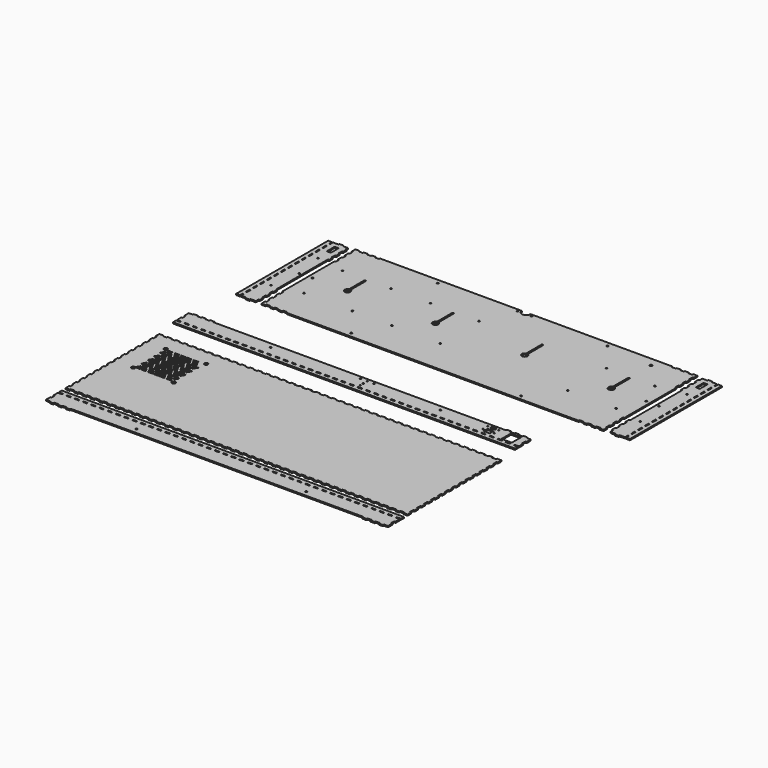
from build123d import *

# Parameters (mm, degrees)
F0_R     = 4.572
F1_DEPTH = 3.175
F0_R_2   = 2.1828252
F0_R_3   = 2.0447
F0_R_4   = 3.175
F0_W     = 2.9972
F0_H     = 11.8654322
F0_R_5   = 2.0828
F0_H_2   = 11.8654068
F0_H_3   = 11.8654576
F0_W_2   = 10.4902
F0_H_4   = 25.4
F0_W_3   = 10.7526836
F0_H_5   = 2.9972
F0_W_4   = 10.7526582
F0_R_6   = 1.5875
F0_W_5   = 16.002
F0_H_6   = 13.3096
F0_R_7   = 1.4224
F0_W_6   = 13.0048
F0_H_7   = 4.699
F0_W_7   = 26.67
F0_H_8   = 30.988


# Not quite as in the source:
# - ends of sketch curves that miss each other by under 0.0002 mm in the source are joined
# - a length typed as a fraction of an inch, garbled in the dataset ("3 / 203.2 mm" for 3/8 in), is restored


with BuildPart() as f1:
    # F0 (on Top) → F1 (new body)
    with BuildSketch(Plane.XY):
        Polygon((-501.14835, -83.3475346), (-511.9010082, -83.3475346), (-511.9010082, -95.2129668), (-508.9038082, -95.2129668), (-508.9038082, -105.8809668), (-511.9010082, -105.8809668), (-511.9010082, -117.746399), (-508.9038082, -117.746399), (-508.9038082, -128.4143736), (-511.9010082, -128.4143736), (-511.9010082, -140.2798058), (-508.9038082, -140.2798058), (-508.9038082, -150.9478058), (-511.9010082, -150.9478058), (-511.9010082, -162.813238), (-508.9038082, -162.813238), (-508.9038082, -173.481238), (-511.9010082, -173.481238), (-511.9010082, -185.3466702), (-508.9038082, -185.3466702), (-508.9038082, -196.0146702), (-511.9010082, -196.0146702), (-511.9010082, -207.8801024), (-508.9038082, -207.8801024), (-508.9038082, -218.5481024), (-511.9010082, -218.5481024), (-511.9010082, -230.4135346), (-508.9038082, -230.4135346), (-508.9038082, -241.0815346), (-511.9010082, -241.0815346), (-511.9010082, -252.9469668), (-508.9038082, -252.9469668), (-508.9038082, -263.6149668), (-511.9010082, -263.6149668), (-511.9010082, -275.4803736), (-508.9038082, -275.4803736), (-508.9038082, -286.1483736), (-511.9010082, -286.1483736), (-511.9010082, -298.0138312), (-508.9038082, -298.0138312), (-508.9038082, -308.6818312), (-511.9010082, -308.6818312), (-511.9010082, -320.547238), (-508.9038082, -320.547238), (-508.9038082, -331.215238), (-511.9010082, -331.215238), (-511.9010082, -343.0806702), (-508.9038082, -343.0806702), (-508.9038082, -353.7486702), (-511.9010082, -353.7486702), (-511.9010082, -365.614077), (-508.9038082, -365.614077), (-508.9038082, -376.282077), (-511.9010082, -376.282077), (-511.9010082, -388.1475346), (-501.14835, -388.1475346), (-501.14835, -385.1503346), (-490.48035, -385.1503346), (-490.48035, -388.1475346), (-479.7276918, -388.1475346), (-479.7276918, -385.1503346), (-469.0596918, -385.1503346), (-469.0596918, -388.1475346), (-458.3070082, -388.1475346), (-458.3070082, -385.1503346), (-447.6390082, -385.1503346), (-447.6390082, -388.1475346), (-436.88635, -388.1475346), (-436.88635, -385.1503346), (-426.21835, -385.1503346), (-426.21835, -388.1475346), (-415.4656918, -388.1475346), (-415.4656918, -385.1503346), (-404.7976918, -385.1503346), (-404.7976918, -388.1475346), (-394.0450082, -388.1475346), (-394.0450082, -385.1503346), (-383.3770082, -385.1503346), (-383.3770082, -388.1475346), (-372.62435, -388.1475346), (-372.62435, -385.1503346), (-361.95635, -385.1503346), (-361.95635, -388.1475346), (-351.2036918, -388.1475346), (-351.2036918, -385.1503346), (-340.5356918, -385.1503346), (-340.5356918, -388.1475346), (-329.7830082, -388.1475346), (-329.7830082, -385.1503346), (-319.1150082, -385.1503346), (-319.1150082, -388.1475346), (-308.36235, -388.1475346), (-308.36235, -385.1503346), (-297.69435, -385.1503346), (-297.69435, -388.1475346), (-286.9416918, -388.1475346), (-286.9416918, -385.1503346), (-276.2736918, -385.1503346), (-276.2736918, -388.1475346), (-265.5210082, -388.1475346), (-265.5210082, -385.1503346), (-254.8530082, -385.1503346), (-254.8530082, -388.1475346), (-244.10035, -388.1475346), (-244.10035, -385.1503346), (-233.43235, -385.1503346), (-233.43235, -388.1475346), (-222.6796918, -388.1475346), (-222.6796918, -385.1503346), (-212.0116918, -385.1503346), (-212.0116918, -388.1475346), (-201.2590082, -388.1475346), (-201.2590082, -385.1503346), (-190.5910082, -385.1503346), (-190.5910082, -388.1475346), (-179.83835, -388.1475346), (-179.83835, -385.1503346), (-169.17035, -385.1503346), (-169.17035, -388.1475346), (-158.4176918, -388.1475346), (-158.4176918, -385.1503346), (-147.7496918, -385.1503346), (-147.7496918, -388.1475346), (-136.9970082, -388.1475346), (-136.9970082, -385.1503346), (-126.3290082, -385.1503346), (-126.3290082, -388.1475346), (-115.57635, -388.1475346), (-115.57635, -385.1503346), (-104.90835, -385.1503346), (-104.90835, -388.1475346), (-94.1556918, -388.1475346), (-94.1556918, -385.1503346), (-83.4876918, -385.1503346), (-83.4876918, -388.1475346), (-72.7350082, -388.1475346), (-72.7350082, -385.1503346), (-62.0670082, -385.1503346), (-62.0670082, -388.1475346), (-51.31435, -388.1475346), (-51.31435, -385.1503346), (-40.64635, -385.1503346), (-40.64635, -388.1475346), (-29.8936918, -388.1475346), (-29.8936918, -385.1503346), (-19.2256918, -385.1503346), (-19.2256918, -388.1475346), (-8.4730082, -388.1475346), (-8.4730082, -385.1503346), (2.1949918, -385.1503346), (2.1949918, -388.1475346), (12.94765, -388.1475346), (12.94765, -385.1503346), (23.61565, -385.1503346), (23.61565, -388.1475346), (34.3683082, -388.1475346), (34.3683082, -385.1503346), (45.0363082, -385.1503346), (45.0363082, -388.1475346), (55.7889918, -388.1475346), (55.7889918, -385.1503346), (66.4569918, -385.1503346), (66.4569918, -388.1475346), (77.20965, -388.1475346), (77.20965, -385.1503346), (87.87765, -385.1503346), (87.87765, -388.1475346), (98.6303082, -388.1475346), (98.6303082, -385.1503346), (109.2983082, -385.1503346), (109.2983082, -388.1475346), (120.0509918, -388.1475346), (120.0509918, -385.1503346), (130.7189918, -385.1503346), (130.7189918, -388.1475346), (141.47165, -388.1475346), (141.47165, -385.1503346), (152.13965, -385.1503346), (152.13965, -388.1475346), (162.8923082, -388.1475346), (162.8923082, -385.1503346), (173.5603082, -385.1503346), (173.5603082, -388.1475346), (184.3129918, -388.1475346), (184.3129918, -385.1503346), (194.9809918, -385.1503346), (194.9809918, -388.1475346), (205.73365, -388.1475346), (205.73365, -385.1503346), (216.40165, -385.1503346), (216.40165, -388.1475346), (227.1543082, -388.1475346), (227.1543082, -385.1503346), (237.8223082, -385.1503346), (237.8223082, -388.1475346), (248.5749918, -388.1475346), (248.5749918, -385.1503346), (259.2429918, -385.1503346), (259.2429918, -388.1475346), (269.99565, -388.1475346), (269.99565, -385.1503346), (280.66365, -385.1503346), (280.66365, -388.1475346), (291.4163082, -388.1475346), (291.4163082, -385.1503346), (302.0843082, -385.1503346), (302.0843082, -388.1475346), (312.8369918, -388.1475346), (312.8369918, -385.1503346), (323.5049918, -385.1503346), (323.5049918, -388.1475346), (334.25765, -388.1475346), (334.25765, -385.1503346), (344.92565, -385.1503346), (344.92565, -388.1475346), (355.6783082, -388.1475346), (355.6783082, -385.1503346), (366.3463082, -385.1503346), (366.3463082, -388.1475346), (377.0989918, -388.1475346), (377.0989918, -376.282077), (374.1017918, -376.282077), (374.1017918, -365.614077), (377.0989918, -365.614077), (377.0989918, -353.7486702), (374.1017918, -353.7486702), (374.1017918, -343.0806702), (377.0989918, -343.0806702), (377.0989918, -331.215238), (374.1017918, -331.215238), (374.1017918, -320.547238), (377.0989918, -320.547238), (377.0989918, -308.6818312), (374.1017918, -308.6818312), (374.1017918, -298.0138312), (377.0989918, -298.0138312), (377.0989918, -286.1483736), (374.1017918, -286.1483736), (374.1017918, -275.4803736), (377.0989918, -275.4803736), (377.0989918, -263.6149668), (374.1017918, -263.6149668), (374.1017918, -252.9469668), (377.0989918, -252.9469668), (377.0989918, -241.0815346), (374.1017918, -241.0815346), (374.1017918, -230.4135346), (377.0989918, -230.4135346), (377.0989918, -218.5481024), (374.1017918, -218.5481024), (374.1017918, -207.8801024), (377.0989918, -207.8801024), (377.0989918, -196.0146702), (374.1017918, -196.0146702), (374.1017918, -185.3466702), (377.0989918, -185.3466702), (377.0989918, -173.481238), (374.1017918, -173.481238), (374.1017918, -162.813238), (377.0989918, -162.813238), (377.0989918, -150.9478058), (374.1017918, -150.9478058), (374.1017918, -140.2798058), (377.0989918, -140.2798058), (377.0989918, -128.4143736), (374.1017918, -128.4143736), (374.1017918, -117.746399), (377.0989918, -117.746399), (377.0989918, -105.8809668), (374.1017918, -105.8809668), (374.1017918, -95.2129668), (377.0989918, -95.2129668), (377.0989918, -83.3475346), (366.3463082, -83.3475346), (366.3463082, -86.3447346), (355.6783082, -86.3447346), (355.6783082, -83.3475346), (344.92565, -83.3475346), (344.92565, -86.3447346), (334.25765, -86.3447346), (334.25765, -83.3475346), (323.5049918, -83.3475346), (323.5049918, -86.3447346), (312.8369918, -86.3447346), (312.8369918, -83.3475346), (302.0843082, -83.3475346), (302.0843082, -86.3447346), (291.4163082, -86.3447346), (291.4163082, -83.3475346), (280.66365, -83.3475346), (280.66365, -86.3447346), (269.99565, -86.3447346), (269.99565, -83.3475346), (259.2429918, -83.3475346), (259.2429918, -86.3447346), (248.5749918, -86.3447346), (248.5749918, -83.3475346), (237.8223082, -83.3475346), (237.8223082, -86.3447346), (227.1543082, -86.3447346), (227.1543082, -83.3475346), (216.40165, -83.3475346), (216.40165, -86.3447346), (205.73365, -86.3447346), (205.73365, -83.3475346), (194.9809918, -83.3475346), (194.9809918, -86.3447346), (184.3129918, -86.3447346), (184.3129918, -83.3475346), (173.5603082, -83.3475346), (173.5603082, -86.3447346), (162.8923082, -86.3447346), (162.8923082, -83.3475346), (152.13965, -83.3475346), (152.13965, -86.3447346), (141.47165, -86.3447346), (141.47165, -83.3475346), (130.7189918, -83.3475346), (130.7189918, -86.3447346), (120.0509918, -86.3447346), (120.0509918, -83.3475346), (109.2983082, -83.3475346), (109.2983082, -86.3447346), (98.6303082, -86.3447346), (98.6303082, -83.3475346), (87.87765, -83.3475346), (87.87765, -86.3447346), (77.20965, -86.3447346), (77.20965, -83.3475346), (66.4569918, -83.3475346), (66.4569918, -86.3447346), (55.7889918, -86.3447346), (55.7889918, -83.3475346), (45.0363082, -83.3475346), (45.0363082, -86.3447346), (34.3683082, -86.3447346), (34.3683082, -83.3475346), (23.61565, -83.3475346), (23.61565, -86.3447346), (12.94765, -86.3447346), (12.94765, -83.3475346), (2.1949918, -83.3475346), (2.1949918, -86.3447346), (-8.4730082, -86.3447346), (-8.4730082, -83.3475346), (-19.2256918, -83.3475346), (-19.2256918, -86.3447346), (-29.8936918, -86.3447346), (-29.8936918, -83.3475346), (-40.64635, -83.3475346), (-40.64635, -86.3447346), (-51.31435, -86.3447346), (-51.31435, -83.3475346), (-62.0670082, -83.3475346), (-62.0670082, -86.3447346), (-72.7350082, -86.3447346), (-72.7350082, -83.3475346), (-83.4876918, -83.3475346), (-83.4876918, -86.3447346), (-94.1556918, -86.3447346), (-94.1556918, -83.3475346), (-104.90835, -83.3475346), (-104.90835, -86.3447346), (-115.57635, -86.3447346), (-115.57635, -83.3475346), (-126.3290082, -83.3475346), (-126.3290082, -86.3447346), (-136.9970082, -86.3447346), (-136.9970082, -83.3475346), (-147.7496918, -83.3475346), (-147.7496918, -86.3447346), (-158.4176918, -86.3447346), (-158.4176918, -83.3475346), (-169.17035, -83.3475346), (-169.17035, -86.3447346), (-179.83835, -86.3447346), (-179.83835, -83.3475346), (-190.5910082, -83.3475346), (-190.5910082, -86.3447346), (-201.2590082, -86.3447346), (-201.2590082, -83.3475346), (-212.0116918, -83.3475346), (-212.0116918, -86.3447346), (-222.6796918, -86.3447346), (-222.6796918, -83.3475346), (-233.43235, -83.3475346), (-233.43235, -86.3447346), (-244.10035, -86.3447346), (-244.10035, -83.3475346), (-254.8530082, -83.3475346), (-254.8530082, -86.3447346), (-265.5210082, -86.3447346), (-265.5210082, -83.3475346), (-276.2736918, -83.3475346), (-276.2736918, -86.3447346), (-286.9416918, -86.3447346), (-286.9416918, -83.3475346), (-297.69435, -83.3475346), (-297.69435, -86.3447346), (-308.36235, -86.3447346), (-308.36235, -83.3475346), (-319.1150082, -83.3475346), (-319.1150082, -86.3447346), (-329.7830082, -86.3447346), (-329.7830082, -83.3475346), (-340.5356918, -83.3475346), (-340.5356918, -86.3447346), (-351.2036918, -86.3447346), (-351.2036918, -83.3475346), (-361.95635, -83.3475346), (-361.95635, -86.3447346), (-372.62435, -86.3447346), (-372.62435, -83.3475346), (-383.3770082, -83.3475346), (-383.3770082, -86.3447346), (-394.0450082, -86.3447346), (-394.0450082, -83.3475346), (-404.7976918, -83.3475346), (-404.7976918, -86.3447346), (-415.4656918, -86.3447346), (-415.4656918, -83.3475346), (-426.21835, -83.3475346), (-426.21835, -86.3447346), (-436.88635, -86.3447346), (-436.88635, -83.3475346), (-447.6390082, -83.3475346), (-447.6390082, -86.3447346), (-458.3070082, -86.3447346), (-458.3070082, -83.3475346), (-469.0596918, -83.3475346), (-469.0596918, -86.3447346), (-479.7276918, -86.3447346), (-479.7276918, -83.3475346), (-490.48035, -83.3475346), (-490.48035, -86.3447346), (-501.14835, -86.3447346), align=None)
        with Locations((-355.68255, -231.9860994)):
            Circle(F0_R, mode=Mode.SUBTRACT)
        with BuildLine():
            ThreePointArc((-457.6334996089, -228.582496957), (-456.511230744, -230.1224381631), (-456.11415, -231.9860994))
            ThreePointArc((-456.11415, -231.9860994), (-464.4699540022, -234.5524219192), (-458.9951698043, -227.7383035036))
            Line((-458.9951698043, -227.7383035036), (-452.8834732, -217.1524994))
            Line((-452.8834732, -217.1524994), (-446.28435, -228.5824994))
            Line((-446.28435, -228.5824994), (-457.6334996089, -228.582496957))
        make_face(mode=Mode.SUBTRACT)
        Polygon((-438.66435, -210.8024994), (-445.2634732, -222.2324994), (-451.862571, -210.8024994), align=None, mode=Mode.SUBTRACT)
        Polygon((-444.242571, -228.5824994), (-437.6434732, -217.1524994), (-431.04435, -228.5824994), align=None, mode=Mode.SUBTRACT)
        Polygon((-420.88435, -210.8024994), (-427.4834732, -222.2324994), (-434.082571, -210.8024994), align=None, mode=Mode.SUBTRACT)
        Polygon((-459.482571, -208.2624994), (-452.8834732, -196.8324994), (-446.28435, -208.2624994), align=None, mode=Mode.SUBTRACT)
        Polygon((-444.242571, -208.2624994), (-437.6434732, -196.8324994), (-431.04435, -208.2624994), align=None, mode=Mode.SUBTRACT)
        Polygon((-426.462571, -228.5824994), (-419.8634732, -217.1524994), (-413.26435, -228.5824994), align=None, mode=Mode.SUBTRACT)
        Polygon((-405.64435, -210.8024994), (-412.2434732, -222.2324994), (-418.842571, -210.8024994), align=None, mode=Mode.SUBTRACT)
        Polygon((-410.9734732, -228.5824994), (-404.37435, -217.1524994), (-397.7752268, -228.5824994), align=None, mode=Mode.SUBTRACT)
        Polygon((-390.1552268, -210.8024994), (-396.75435, -222.2324994), (-403.3534732, -210.8024994), align=None, mode=Mode.SUBTRACT)
        Polygon((-426.462571, -208.2624994), (-419.8634732, -196.8324994), (-413.26435, -208.2624994), align=None, mode=Mode.SUBTRACT)
        Polygon((-410.9734732, -208.2624994), (-404.37435, -196.8324994), (-397.7752268, -208.2624994), align=None, mode=Mode.SUBTRACT)
        Polygon((-438.66435, -190.4824994), (-445.2634732, -201.9124994), (-451.862571, -190.4824994), align=None, mode=Mode.SUBTRACT)
        Polygon((-420.88435, -190.4824994), (-427.4834732, -201.9124994), (-434.082571, -190.4824994), align=None, mode=Mode.SUBTRACT)
        Polygon((-459.482571, -187.9424994), (-452.8834732, -176.5124994), (-446.28435, -187.9424994), align=None, mode=Mode.SUBTRACT)
        Polygon((-438.66435, -170.1624994), (-445.2634732, -181.5924994), (-451.862571, -170.1624994), align=None, mode=Mode.SUBTRACT)
        Polygon((-444.242571, -187.9424994), (-437.6434732, -176.5124994), (-431.04435, -187.9424994), align=None, mode=Mode.SUBTRACT)
        Polygon((-420.88435, -170.1624994), (-427.4834732, -181.5924994), (-434.082571, -170.1624994), align=None, mode=Mode.SUBTRACT)
        Polygon((-405.64435, -190.4824994), (-412.2434732, -201.9124994), (-418.842571, -190.4824994), align=None, mode=Mode.SUBTRACT)
        Polygon((-390.1552268, -190.4824994), (-396.75435, -201.9124994), (-403.3534732, -190.4824994), align=None, mode=Mode.SUBTRACT)
        Polygon((-426.462571, -187.9424994), (-419.8634732, -176.5124994), (-413.26435, -187.9424994), align=None, mode=Mode.SUBTRACT)
        Polygon((-405.64435, -170.1624994), (-412.2434732, -181.5924994), (-418.842571, -170.1624994), align=None, mode=Mode.SUBTRACT)
        Polygon((-410.9734732, -187.9424994), (-404.37435, -176.5124994), (-397.7752268, -187.9424994), align=None, mode=Mode.SUBTRACT)
        Polygon((-390.1552268, -170.1624994), (-396.75435, -181.5924994), (-403.3534732, -170.1624994), align=None, mode=Mode.SUBTRACT)
        with Locations((-460.68615, -126.9824994)):
            Circle(F0_R, mode=Mode.SUBTRACT)
        Polygon((-459.482571, -167.6224994), (-452.8834732, -156.1924994), (-446.28435, -167.6224994), align=None, mode=Mode.SUBTRACT)
        Polygon((-444.242571, -167.6224994), (-437.6434732, -156.1924994), (-431.04435, -167.6224994), align=None, mode=Mode.SUBTRACT)
        Polygon((-438.66435, -149.8424994), (-445.2634732, -161.2724994), (-451.862571, -149.8424994), align=None, mode=Mode.SUBTRACT)
        Polygon((-420.88435, -149.8424994), (-427.4834732, -161.2724994), (-434.082571, -149.8424994), align=None, mode=Mode.SUBTRACT)
        Polygon((-426.462571, -167.6224994), (-419.8634732, -156.1924994), (-413.26435, -167.6224994), align=None, mode=Mode.SUBTRACT)
        Polygon((-410.9734732, -167.6224994), (-404.37435, -156.1924994), (-397.7752268, -167.6224994), align=None, mode=Mode.SUBTRACT)
        Polygon((-405.64435, -149.8424994), (-412.2434732, -161.2724994), (-418.842571, -149.8424994), align=None, mode=Mode.SUBTRACT)
        Polygon((-390.1552268, -149.8424994), (-396.75435, -161.2724994), (-403.3534732, -149.8424994), align=None, mode=Mode.SUBTRACT)
        Polygon((-459.482571, -147.3024994), (-452.8834732, -135.8724994), (-446.28435, -147.3024994), align=None, mode=Mode.SUBTRACT)
        Polygon((-438.66435, -129.5224994), (-445.2634732, -140.9524994), (-451.862571, -129.5224994), align=None, mode=Mode.SUBTRACT)
        Polygon((-444.242571, -147.3024994), (-437.6434732, -135.8724994), (-431.04435, -147.3024994), align=None, mode=Mode.SUBTRACT)
        Polygon((-420.88435, -129.5224994), (-427.4834732, -140.9524994), (-434.082571, -129.5224994), align=None, mode=Mode.SUBTRACT)
        Polygon((-426.462571, -147.3024994), (-419.8634732, -135.8724994), (-413.26435, -147.3024994), align=None, mode=Mode.SUBTRACT)
        Polygon((-405.64435, -129.5224994), (-412.2434732, -140.9524994), (-418.842571, -129.5224994), align=None, mode=Mode.SUBTRACT)
        Polygon((-410.9734732, -147.3024994), (-404.37435, -135.8724994), (-397.7752268, -147.3024994), align=None, mode=Mode.SUBTRACT)
        Polygon((-390.1552268, -129.5224994), (-396.75435, -140.9524994), (-403.3534732, -129.5224994), align=None, mode=Mode.SUBTRACT)
        Polygon((-395.7334732, -228.5824994), (-389.13435, -217.1524994), (-382.5352268, -228.5824994), align=None, mode=Mode.SUBTRACT)
        Polygon((-372.3752268, -210.8024994), (-378.97435, -222.2324994), (-385.5734732, -210.8024994), align=None, mode=Mode.SUBTRACT)
        Polygon((-377.9534732, -228.5824994), (-371.35435, -217.1524994), (-364.7552268, -228.5824994), align=None, mode=Mode.SUBTRACT)
        Polygon((-357.1352268, -210.8024994), (-363.73435, -222.2324994), (-370.3334732, -210.8024994), align=None, mode=Mode.SUBTRACT)
        Polygon((-395.7334732, -208.2624994), (-389.13435, -196.8324994), (-382.5352268, -208.2624994), align=None, mode=Mode.SUBTRACT)
        Polygon((-377.9534732, -208.2624994), (-371.35435, -196.8324994), (-364.7552268, -208.2624994), align=None, mode=Mode.SUBTRACT)
        Polygon((-372.3752268, -190.4824994), (-378.97435, -201.9124994), (-385.5734732, -190.4824994), align=None, mode=Mode.SUBTRACT)
        Polygon((-357.1352268, -190.4824994), (-363.73435, -201.9124994), (-370.3334732, -190.4824994), align=None, mode=Mode.SUBTRACT)
        Polygon((-395.7334732, -187.9424994), (-389.13435, -176.5124994), (-382.5352268, -187.9424994), align=None, mode=Mode.SUBTRACT)
        Polygon((-372.3752268, -170.1624994), (-378.97435, -181.5924994), (-385.5734732, -170.1624994), align=None, mode=Mode.SUBTRACT)
        Polygon((-377.9534732, -187.9424994), (-371.35435, -176.5124994), (-364.7552268, -187.9424994), align=None, mode=Mode.SUBTRACT)
        Polygon((-357.1352268, -170.1624994), (-363.73435, -181.5924994), (-370.3334732, -170.1624994), align=None, mode=Mode.SUBTRACT)
        Polygon((-395.7334732, -167.6224994), (-389.13435, -156.1924994), (-382.5352268, -167.6224994), align=None, mode=Mode.SUBTRACT)
        Polygon((-377.9534732, -167.6224994), (-371.35435, -156.1924994), (-364.7552268, -167.6224994), align=None, mode=Mode.SUBTRACT)
        Polygon((-372.3752268, -149.8424994), (-378.97435, -161.2724994), (-385.5734732, -149.8424994), align=None, mode=Mode.SUBTRACT)
        Polygon((-357.1352268, -149.8424994), (-363.73435, -161.2724994), (-370.3334732, -149.8424994), align=None, mode=Mode.SUBTRACT)
        Polygon((-395.7334732, -147.3024994), (-389.13435, -135.8724994), (-382.5352268, -147.3024994), align=None, mode=Mode.SUBTRACT)
        Polygon((-372.3752268, -129.5224994), (-378.97435, -140.9524994), (-385.5734732, -129.5224994), align=None, mode=Mode.SUBTRACT)
        Polygon((-377.9534732, -147.3024994), (-371.35435, -135.8724994), (-364.7552268, -147.3024994), align=None, mode=Mode.SUBTRACT)
        with BuildLine():
            ThreePointArc((-357.958210521, -130.9479190743), (-357.9737139071, -123.0260171302), (-351.11055, -126.9824994))
            ThreePointArc((-351.11055, -126.9824994), (-353.3913860929, -130.9389816698), (-357.958210521, -130.9479190743))
        make_face(mode=Mode.SUBTRACT)
    extrude(amount=F1_DEPTH)


with BuildPart() as f1b:
    # F0 (on Top) → F1, piece 2 (new body)
    with BuildSketch(Plane.XY):
        with BuildLine():
            Line((-369.32235, 150.7120684), (-358.5696664, 150.7120684))
            Line((-358.5696664, 150.7120684), (380.4009918, 150.7120684))
            Line((380.4009918, 150.7120684), (391.15365, 150.7120684))
            Line((391.15365, 150.7120684), (391.15365, 153.7092684))
            Line((391.15365, 153.7092684), (401.82165, 153.7092684))
            Line((401.82165, 153.7092684), (401.82165, 150.7120684))
            Line((401.82165, 150.7120684), (412.5743336, 150.7120684))
            Line((412.5743336, 150.7120684), (412.5743336, 153.7092684))
            Line((412.5743336, 153.7092684), (423.2423336, 153.7092684))
            Line((423.2423336, 153.7092684), (423.2423336, 150.7120684))
            Line((423.2423336, 150.7120684), (433.9949918, 150.7120684))
            Line((433.9949918, 150.7120684), (433.9949918, 153.7092684))
            Line((433.9949918, 153.7092684), (444.6629918, 153.7092684))
            Line((444.6629918, 153.7092684), (444.6629918, 150.7120684))
            Line((444.6629918, 150.7120684), (455.41565, 150.7120684))
            Line((455.41565, 150.7120684), (455.41565, 162.5775006))
            Line((455.41565, 162.5775006), (452.41845, 162.5775006))
            Line((452.41845, 162.5775006), (452.41845, 173.2455006))
            Line((452.41845, 173.2455006), (455.41565, 173.2455006))
            Line((455.41565, 173.2455006), (455.41565, 185.1109074))
            Line((455.41565, 185.1109074), (452.41845, 185.1109074))
            Line((452.41845, 185.1109074), (452.41845, 195.7789074))
            Line((452.41845, 195.7789074), (455.41565, 195.7789074))
            Line((455.41565, 195.7789074), (455.41565, 207.644365))
            Line((455.41565, 207.644365), (452.41845, 207.644365))
            Line((452.41845, 207.644365), (452.41845, 218.312365))
            Line((452.41845, 218.312365), (455.41565, 218.312365))
            Line((455.41565, 218.312365), (455.41565, 387.9117718))
            Line((455.41565, 387.9117718), (452.41845, 387.9117718))
            Line((452.41845, 387.9117718), (452.41845, 398.5797718))
            Line((452.41845, 398.5797718), (455.41565, 398.5797718))
            Line((455.41565, 398.5797718), (455.41565, 410.445204))
            Line((455.41565, 410.445204), (452.41845, 410.445204))
            Line((452.41845, 410.445204), (452.41845, 421.113204))
            Line((452.41845, 421.113204), (455.41565, 421.113204))
            Line((455.41565, 421.113204), (455.41565, 432.9786362))
            Line((455.41565, 432.9786362), (452.41845, 432.9786362))
            Line((452.41845, 432.9786362), (452.41845, 443.6466362))
            Line((452.41845, 443.6466362), (455.41565, 443.6466362))
            Line((455.41565, 443.6466362), (455.41565, 455.5120684))
            Line((455.41565, 455.5120684), (444.6629918, 455.5120684))
            Line((444.6629918, 455.5120684), (444.6629918, 452.5148684))
            Line((444.6629918, 452.5148684), (433.9949918, 452.5148684))
            Line((433.9949918, 452.5148684), (433.9949918, 455.5120684))
            Line((433.9949918, 455.5120684), (423.2423336, 455.5120684))
            Line((423.2423336, 455.5120684), (423.2423336, 452.5148684))
            Line((423.2423336, 452.5148684), (412.5743336, 452.5148684))
            Line((412.5743336, 452.5148684), (412.5743336, 455.5120684))
            Line((412.5743336, 455.5120684), (401.82165, 455.5120684))
            Line((401.82165, 455.5120684), (401.82165, 452.5148684))
            Line((401.82165, 452.5148684), (391.15365, 452.5148684))
            Line((391.15365, 452.5148684), (391.15365, 455.5120684))
            Line((391.15365, 455.5120684), (380.4009918, 455.5120684))
            Line((380.4009918, 455.5120684), (22.3456754, 455.5120684))
            ThreePointArc((22.3456754, 455.5120684), (10.91565, 444.0820684), (-0.51435, 455.5120684))
            Line((-0.51435, 455.5120684), (-358.5696664, 455.5120684))
            Line((-358.5696664, 455.5120684), (-369.32235, 455.5120684))
            Line((-369.32235, 455.5120684), (-369.32235, 452.5148684))
            Line((-369.32235, 452.5148684), (-379.99035, 452.5148684))
            Line((-379.99035, 452.5148684), (-379.99035, 455.5120684))
            Line((-379.99035, 455.5120684), (-390.7430082, 455.5120684))
            Line((-390.7430082, 455.5120684), (-390.7430082, 452.5148684))
            Line((-390.7430082, 452.5148684), (-401.4110082, 452.5148684))
            Line((-401.4110082, 452.5148684), (-401.4110082, 455.5120684))
            Line((-401.4110082, 455.5120684), (-412.1636664, 455.5120684))
            Line((-412.1636664, 455.5120684), (-412.1636664, 452.5148684))
            Line((-412.1636664, 452.5148684), (-422.8316664, 452.5148684))
            Line((-422.8316664, 452.5148684), (-422.8316664, 455.5120684))
            Line((-422.8316664, 455.5120684), (-433.58435, 455.5120684))
            Line((-433.58435, 455.5120684), (-433.58435, 443.6466362))
            Line((-433.58435, 443.6466362), (-430.58715, 443.6466362))
            Line((-430.58715, 443.6466362), (-430.58715, 432.9786362))
            Line((-430.58715, 432.9786362), (-433.58435, 432.9786362))
            Line((-433.58435, 432.9786362), (-433.58435, 421.113204))
            Line((-433.58435, 421.113204), (-430.58715, 421.113204))
            Line((-430.58715, 421.113204), (-430.58715, 410.445204))
            Line((-430.58715, 410.445204), (-433.58435, 410.445204))
            Line((-433.58435, 410.445204), (-433.58435, 398.5797718))
            Line((-433.58435, 398.5797718), (-430.58715, 398.5797718))
            Line((-430.58715, 398.5797718), (-430.58715, 387.9117718))
            Line((-430.58715, 387.9117718), (-433.58435, 387.9117718))
            Line((-433.58435, 387.9117718), (-433.58435, 218.312365))
            Line((-433.58435, 218.312365), (-430.58715, 218.312365))
            Line((-430.58715, 218.312365), (-430.58715, 207.644365))
            Line((-430.58715, 207.644365), (-433.58435, 207.644365))
            Line((-433.58435, 207.644365), (-433.58435, 195.7789074))
            Line((-433.58435, 195.7789074), (-430.58715, 195.7789074))
            Line((-430.58715, 195.7789074), (-430.58715, 185.1109074))
            Line((-430.58715, 185.1109074), (-433.58435, 185.1109074))
            Line((-433.58435, 185.1109074), (-433.58435, 173.2455006))
            Line((-433.58435, 173.2455006), (-430.58715, 173.2455006))
            Line((-430.58715, 173.2455006), (-430.58715, 162.5775006))
            Line((-430.58715, 162.5775006), (-433.58435, 162.5775006))
            Line((-433.58435, 162.5775006), (-433.58435, 150.7120684))
            Line((-433.58435, 150.7120684), (-422.8316664, 150.7120684))
            Line((-422.8316664, 150.7120684), (-422.8316664, 153.7092684))
            Line((-422.8316664, 153.7092684), (-412.1636664, 153.7092684))
            Line((-412.1636664, 153.7092684), (-412.1636664, 150.7120684))
            Line((-412.1636664, 150.7120684), (-401.4110082, 150.7120684))
            Line((-401.4110082, 150.7120684), (-401.4110082, 153.7092684))
            Line((-401.4110082, 153.7092684), (-390.7430082, 153.7092684))
            Line((-390.7430082, 153.7092684), (-390.7430082, 150.7120684))
            Line((-390.7430082, 150.7120684), (-379.99035, 150.7120684))
            Line((-379.99035, 150.7120684), (-379.99035, 153.7092684))
            Line((-379.99035, 153.7092684), (-369.32235, 153.7092684))
            Line((-369.32235, 153.7092684), (-369.32235, 150.7120684))
        make_face()
        with Locations((-209.83575, 162.5739446)):
            Circle(F0_R_2, mode=Mode.SUBTRACT)
        with Locations((-394.846175, 240.2502434)):
            Circle(F0_R_3, mode=Mode.SUBTRACT)
        with Locations((-422.8316664, 303.1120684)):
            Circle(F0_R_2, mode=Mode.SUBTRACT)
        with Locations((-269.122525, 240.2502434)):
            Circle(F0_R_3, mode=Mode.SUBTRACT)
        with BuildLine():
            ThreePointArc((-329.8253469107, 310.4198112567), (-331.98435, 295.4920684), (-334.1433530893, 310.4198112567))
            Line((-334.1433530893, 310.4198112567), (-334.14335, 360.6975006))
            ThreePointArc((-334.14335, 360.6975006), (-331.98435, 361.5320684), (-329.8253483574, 360.6975024072))
            Line((-329.8253483574, 360.6975024072), (-329.8253469107, 310.4198112567))
        make_face(mode=Mode.SUBTRACT)
        with Locations((-394.846175, 365.9738934)):
            Circle(F0_R_3, mode=Mode.SUBTRACT)
        with Locations((-269.122525, 365.9738934)):
            Circle(F0_R_3, mode=Mode.SUBTRACT)
        with Locations((-166.246175, 240.2502434)):
            Circle(F0_R_3, mode=Mode.SUBTRACT)
        with Locations((-40.522525, 240.2502434)):
            Circle(F0_R_3, mode=Mode.SUBTRACT)
        with BuildLine():
            ThreePointArc((-101.2253469107, 310.4198112567), (-103.38435, 295.4920684), (-105.5433530893, 310.4198112567))
            Line((-105.5433530893, 310.4198112567), (-105.54335, 360.6975006))
            ThreePointArc((-105.54335, 360.6975006), (-103.38435, 361.5320684), (-101.2253483574, 360.6975024072))
            Line((-101.2253483574, 360.6975024072), (-101.2253469107, 310.4198112567))
        make_face(mode=Mode.SUBTRACT)
        with Locations((-166.246175, 365.9738934)):
            Circle(F0_R_3, mode=Mode.SUBTRACT)
        with Locations((-209.83575, 443.6466362)):
            Circle(F0_R_2, mode=Mode.SUBTRACT)
        with Locations((-40.522525, 365.9738934)):
            Circle(F0_R_3, mode=Mode.SUBTRACT)
        with Locations((-6.86435, 449.5975006)):
            Circle(F0_R_2, mode=Mode.SUBTRACT)
        with Locations((231.66705, 162.5739446)):
            Circle(F0_R_2, mode=Mode.SUBTRACT)
        with BuildLine():
            ThreePointArc((127.3746784893, 314.8616362567), (125.2156754, 299.9338934), (123.0566723107, 314.8616362567))
            Line((123.0566723107, 314.8616362567), (123.0566754, 365.1393256))
            ThreePointArc((123.0566754, 365.1393256), (125.2156754, 365.9738934), (127.3746770426, 365.1393274072))
            Line((127.3746770426, 365.1393274072), (127.3746784893, 314.8616362567))
        make_face(mode=Mode.SUBTRACT)
        with Locations((28.69565, 449.5975006)):
            Circle(F0_R_2, mode=Mode.SUBTRACT)
        with Locations((231.66705, 443.6466362)):
            Circle(F0_R_2, mode=Mode.SUBTRACT)
        with Locations((290.953825, 240.2502434)):
            Circle(F0_R_3, mode=Mode.SUBTRACT)
        with BuildLine():
            ThreePointArc((355.9746530893, 310.4198112567), (353.81565, 295.4920684), (351.6566469107, 310.4198112567))
            Line((351.6566469107, 310.4198112567), (351.65665, 360.6975006))
            ThreePointArc((351.65665, 360.6975006), (353.81565, 361.5320684), (355.9746516426, 360.6975024072))
            Line((355.9746516426, 360.6975024072), (355.9746530893, 310.4198112567))
        make_face(mode=Mode.SUBTRACT)
        with Locations((416.677475, 240.2502434)):
            Circle(F0_R_3, mode=Mode.SUBTRACT)
        with Locations((444.6409446, 303.101121)):
            Circle(F0_R_2, mode=Mode.SUBTRACT)
        with Locations((290.953825, 365.9738934)):
            Circle(F0_R_3, mode=Mode.SUBTRACT)
        with Locations((353.81565, 431.8175006)):
            Circle(F0_R_4, mode=Mode.SUBTRACT)
        with Locations((416.677475, 365.9738934)):
            Circle(F0_R_3, mode=Mode.SUBTRACT)
    extrude(amount=F1_DEPTH)


with BuildPart() as f1c:
    # F0 (on Top) → F1, piece 3 (new body)
    with BuildSketch(Plane.XY):
        Polygon((-446.28435, 216.6432294), (-449.28155, 216.6432294), (-449.28155, 386.2426616), (-446.28435, 386.2426616), (-446.28435, 396.9106616), (-449.28155, 396.9106616), (-449.28155, 408.7760938), (-446.28435, 408.7760938), (-446.28435, 419.4440938), (-449.28155, 419.4440938), (-449.28155, 431.3095006), (-446.28435, 431.3095006), (-446.28435, 441.9775006), (-449.28155, 441.9775006), (-449.28155, 450.8457582), (-463.17535, 450.8457582), (-463.17535, 453.8429582), (-473.84335, 453.8429582), (-473.84335, 450.8457582), (-487.73715, 450.8457582), (-487.73715, 441.9775006), (-490.73435, 441.9775006), (-490.73435, 450.8457582), (-500.43715, 450.8457582), (-500.43715, 152.0401582), (-490.73435, 152.0401582), (-490.73435, 160.9083904), (-487.73715, 160.9083904), (-487.73715, 152.0401582), (-473.84335, 152.0401582), (-473.84335, 149.0429582), (-463.17535, 149.0429582), (-463.17535, 152.0401582), (-449.28155, 152.0401582), (-449.28155, 160.9083904), (-446.28435, 160.9083904), (-446.28435, 171.5763904), (-449.28155, 171.5763904), (-449.28155, 183.4418226), (-446.28435, 183.4418226), (-446.28435, 194.1097972), (-449.28155, 194.1097972), (-449.28155, 205.9752294), (-446.28435, 205.9752294), align=None)
        with Locations((-489.23575, 177.5091065)):
            Rectangle(F0_W, F0_H, mode=Mode.SUBTRACT)
        with Locations((-489.23575, 200.0425133)):
            Rectangle(F0_W, F0_H, mode=Mode.SUBTRACT)
        with Locations((-489.23575, 222.5759455)):
            Rectangle(F0_W, F0_H, mode=Mode.SUBTRACT)
        with Locations((-468.50935, 225.2429582)):
            Circle(F0_R_5, mode=Mode.SUBTRACT)
        with Locations((-489.23575, 245.1093777)):
            Rectangle(F0_W, F0_H, mode=Mode.SUBTRACT)
        with Locations((-489.23575, 267.6428099)):
            Rectangle(F0_W, F0_H, mode=Mode.SUBTRACT)
        with Locations((-489.23575, 290.1762421)):
            Rectangle(F0_W, F0_H, mode=Mode.SUBTRACT)
        with Locations((-489.23575, 312.7096743)):
            Rectangle(F0_W, F0_H, mode=Mode.SUBTRACT)
        with Locations((-489.23575, 335.2430938)):
            Rectangle(F0_W, F0_H_2, mode=Mode.SUBTRACT)
        with Locations((-456.22845, 301.4429582)):
            Circle(F0_R_2, mode=Mode.SUBTRACT)
        with Locations((-489.23575, 357.776526)):
            Rectangle(F0_W, F0_H_3, mode=Mode.SUBTRACT)
        with Locations((-489.23575, 380.3099582)):
            Rectangle(F0_W, F0_H_2, mode=Mode.SUBTRACT)
        with Locations((-468.50935, 377.6429582)):
            Circle(F0_R_5, mode=Mode.SUBTRACT)
        with Locations((-489.23575, 402.8433777)):
            Rectangle(F0_W, F0_H, mode=Mode.SUBTRACT)
        with Locations((-489.23575, 425.3767972)):
            Rectangle(F0_W, F0_H_2, mode=Mode.SUBTRACT)
        with Locations((-468.34425, 425.3767972)):
            Rectangle(F0_W_2, F0_H_4, mode=Mode.SUBTRACT)
    extrude(amount=F1_DEPTH)


with BuildPart() as f1d:
    # F0 (on Top) → F1, piece 4 (new body)
    with BuildSketch(Plane.XY):
        Polygon((302.25365, 25.4175006), (-458.22235, 25.4175006), (-458.22235, 28.4147006), (-468.89035, 28.4147006), (-468.89035, 25.4175006), (-479.6430082, 25.4175006), (-479.6430082, 28.4147006), (-490.3110082, 28.4147006), (-490.3110082, 25.4175006), (-501.0636918, 25.4175006), (-501.0636918, 28.4147006), (-511.7316918, 28.4147006), (-511.7316918, 25.4175006), (-522.48435, 25.4175006), (-522.48435, 11.5237006), (-519.48715, 11.5237006), (-519.48715, 0.8557006), (-522.48435, 0.8557006), (-522.48435, -13.0380994), (-511.7316918, -13.0380994), (-511.7316918, -16.0352994), (-522.48435, -16.0352994), (-522.48435, -25.7380994), (366.51565, -25.7380994), (366.51565, -16.0352994), (355.7629918, -16.0352994), (355.7629918, -13.0380994), (366.51565, -13.0380994), (366.51565, 0.8557006), (363.51845, 0.8557006), (363.51845, 11.5237006), (366.51565, 11.5237006), (366.51565, 25.4175006), (355.7629918, 25.4175006), (355.7629918, 28.4147006), (345.0949918, 28.4147006), (345.0949918, 25.4175006), (334.3423082, 25.4175006), (334.3423082, 28.4147006), (323.6743082, 28.4147006), (323.6743082, 25.4175006), (312.92165, 25.4175006), (312.92165, 28.4147006), (302.25365, 28.4147006), align=None)
        with Locations((-495.68735, -14.5366994)):
            Rectangle(F0_W_3, F0_H_5, mode=Mode.SUBTRACT)
        with Locations((-474.2666791, -14.5366994)):
            Rectangle(F0_W_4, F0_H_5, mode=Mode.SUBTRACT)
        with Locations((-452.8460209, -14.5366994)):
            Rectangle(F0_W_4, F0_H_5, mode=Mode.SUBTRACT)
        with Locations((-431.42535, -14.5366994)):
            Rectangle(F0_W_3, F0_H_5, mode=Mode.SUBTRACT)
        with Locations((-410.0046791, -14.5366994)):
            Rectangle(F0_W_4, F0_H_5, mode=Mode.SUBTRACT)
        with Locations((-388.5840209, -14.5366994)):
            Rectangle(F0_W_4, F0_H_5, mode=Mode.SUBTRACT)
        with Locations((-367.16335, -14.5366994)):
            Rectangle(F0_W_3, F0_H_5, mode=Mode.SUBTRACT)
        with Locations((-345.7426791, -14.5366994)):
            Rectangle(F0_W_4, F0_H_5, mode=Mode.SUBTRACT)
        with Locations((-324.3220209, -14.5366994)):
            Rectangle(F0_W_4, F0_H_5, mode=Mode.SUBTRACT)
        with Locations((-302.90135, -14.5366994)):
            Rectangle(F0_W_3, F0_H_5, mode=Mode.SUBTRACT)
        with Locations((-281.4806791, -14.5366994)):
            Rectangle(F0_W_4, F0_H_5, mode=Mode.SUBTRACT)
        with Locations((-260.0600209, -14.5366994)):
            Rectangle(F0_W_4, F0_H_5, mode=Mode.SUBTRACT)
        with Locations((-238.63935, -14.5366994)):
            Rectangle(F0_W_3, F0_H_5, mode=Mode.SUBTRACT)
        with Locations((-217.2186791, -14.5366994)):
            Rectangle(F0_W_4, F0_H_5, mode=Mode.SUBTRACT)
        with Locations((-195.7980209, -14.5366994)):
            Rectangle(F0_W_4, F0_H_5, mode=Mode.SUBTRACT)
        with Locations((-174.37735, -14.5366994)):
            Rectangle(F0_W_3, F0_H_5, mode=Mode.SUBTRACT)
        with Locations((-152.9566791, -14.5366994)):
            Rectangle(F0_W_4, F0_H_5, mode=Mode.SUBTRACT)
        with Locations((-131.5360209, -14.5366994)):
            Rectangle(F0_W_4, F0_H_5, mode=Mode.SUBTRACT)
        with Locations((-110.11535, -14.5366994)):
            Rectangle(F0_W_3, F0_H_5, mode=Mode.SUBTRACT)
        with Locations((-88.6946791, -14.5366994)):
            Rectangle(F0_W_4, F0_H_5, mode=Mode.SUBTRACT)
        with Locations((-67.2740209, -14.5366994)):
            Rectangle(F0_W_4, F0_H_5, mode=Mode.SUBTRACT)
        with Locations((-45.85335, -14.5366994)):
            Rectangle(F0_W_3, F0_H_5, mode=Mode.SUBTRACT)
        with Locations((-52.58435, -5.0624994)):
            Circle(F0_R_6, mode=Mode.SUBTRACT)
        with Locations((-24.4326791, -14.5366994)):
            Rectangle(F0_W_4, F0_H_5, mode=Mode.SUBTRACT)
        with Locations((-3.0120209, -14.5366994)):
            Rectangle(F0_W_4, F0_H_5, mode=Mode.SUBTRACT)
        with Locations((18.40865, -14.5366994)):
            Rectangle(F0_W_3, F0_H_5, mode=Mode.SUBTRACT)
        with Locations((39.8293209, -14.5366994)):
            Rectangle(F0_W_4, F0_H_5, mode=Mode.SUBTRACT)
        with Locations((61.2499791, -14.5366994)):
            Rectangle(F0_W_4, F0_H_5, mode=Mode.SUBTRACT)
        with Locations((82.67065, -14.5366994)):
            Rectangle(F0_W_3, F0_H_5, mode=Mode.SUBTRACT)
        with Locations((104.0913209, -14.5366994)):
            Rectangle(F0_W_4, F0_H_5, mode=Mode.SUBTRACT)
        with Locations((125.5119791, -14.5366994)):
            Rectangle(F0_W_4, F0_H_5, mode=Mode.SUBTRACT)
        with Locations((146.93265, -14.5366994)):
            Rectangle(F0_W_3, F0_H_5, mode=Mode.SUBTRACT)
        with Locations((168.3533209, -14.5366994)):
            Rectangle(F0_W_4, F0_H_5, mode=Mode.SUBTRACT)
        with Locations((189.7739791, -14.5366994)):
            Rectangle(F0_W_4, F0_H_5, mode=Mode.SUBTRACT)
        with Locations((211.19465, -14.5366994)):
            Rectangle(F0_W_3, F0_H_5, mode=Mode.SUBTRACT)
        with Locations((232.6153209, -14.5366994)):
            Rectangle(F0_W_4, F0_H_5, mode=Mode.SUBTRACT)
        with Locations((254.0359791, -14.5366994)):
            Rectangle(F0_W_4, F0_H_5, mode=Mode.SUBTRACT)
        with Locations((275.45665, -14.5366994)):
            Rectangle(F0_W_3, F0_H_5, mode=Mode.SUBTRACT)
        with Locations((296.8773209, -14.5366994)):
            Rectangle(F0_W_4, F0_H_5, mode=Mode.SUBTRACT)
        with Locations((318.2979791, -14.5366994)):
            Rectangle(F0_W_4, F0_H_5, mode=Mode.SUBTRACT)
        with Locations((339.71865, -14.5366994)):
            Rectangle(F0_W_3, F0_H_5, mode=Mode.SUBTRACT)
        with Locations((-298.73575, 11.5237006)):
            Circle(F0_R_2, mode=Mode.SUBTRACT)
        with Locations((-70.36435, 17.7975006)):
            Circle(F0_R_2, mode=Mode.SUBTRACT)
        with Locations((-52.58435, 5.0975006)):
            Circle(F0_R_6, mode=Mode.SUBTRACT)
        with Locations((-52.58435, 17.7975006)):
            Circle(F0_R_6, mode=Mode.SUBTRACT)
        with Locations((-34.80435, 17.7975006)):
            Circle(F0_R_2, mode=Mode.SUBTRACT)
        with Locations((142.76705, 11.5237006)):
            Circle(F0_R_2, mode=Mode.SUBTRACT)
        with Locations((262.56615, 0.8557006)):
            Circle(F0_R_6, mode=Mode.SUBTRACT)
        with Locations((276.85365, 0.8557006)):
            Rectangle(F0_W_5, F0_H_6, mode=Mode.SUBTRACT)
        with Locations((291.14115, 0.8557006)):
            Circle(F0_R_6, mode=Mode.SUBTRACT)
        with Locations((262.56615, 16.0957006)):
            Circle(F0_R_7, mode=Mode.SUBTRACT)
        with Locations((276.85365, 16.0957006)):
            Rectangle(F0_W_6, F0_H_7, mode=Mode.SUBTRACT)
        with Locations((291.14115, 16.0957006)):
            Circle(F0_R_7, mode=Mode.SUBTRACT)
        with Locations((331.9365472, 5.6893968)):
            Rectangle(F0_W_7, F0_H_8, mode=Mode.SUBTRACT)
    extrude(amount=F1_DEPTH)


with BuildPart() as f1e:
    # F0 (on Top) → F1, piece 5 (new body)
    with BuildSketch(Plane.XY):
        Polygon((-446.8459948, -452.5148684), (313.6300052, -452.5148684), (313.6300052, -455.5120684), (324.2980052, -455.5120684), (324.2980052, -452.5148684), (335.0506634, -452.5148684), (335.0506634, -455.5120684), (345.7186634, -455.5120684), (345.7186634, -452.5148684), (356.471347, -452.5148684), (356.471347, -455.5120684), (367.139347, -455.5120684), (367.139347, -452.5148684), (377.8920052, -452.5148684), (377.8920052, -438.6210684), (374.8948052, -438.6210684), (374.8948052, -427.9530684), (377.8920052, -427.9530684), (377.8920052, -414.0592684), (367.139347, -414.0592684), (367.139347, -411.0620684), (377.8920052, -411.0620684), (377.8920052, -401.3592684), (-511.1079948, -401.3592684), (-511.1079948, -411.0620684), (-500.3553366, -411.0620684), (-500.3553366, -414.0592684), (-511.1079948, -414.0592684), (-511.1079948, -427.9530684), (-508.1107948, -427.9530684), (-508.1107948, -438.6210684), (-511.1079948, -438.6210684), (-511.1079948, -452.5148684), (-500.3553366, -452.5148684), (-500.3553366, -455.5120684), (-489.6873366, -455.5120684), (-489.6873366, -452.5148684), (-478.934653, -452.5148684), (-478.934653, -455.5120684), (-468.266653, -455.5120684), (-468.266653, -452.5148684), (-457.5139948, -452.5148684), (-457.5139948, -455.5120684), (-446.8459948, -455.5120684), align=None)
        with Locations((-484.3109948, -412.5606684)):
            Rectangle(F0_W_3, F0_H_5, mode=Mode.SUBTRACT)
        with Locations((-462.8903239, -412.5606684)):
            Rectangle(F0_W_4, F0_H_5, mode=Mode.SUBTRACT)
        with Locations((-441.4696657, -412.5606684)):
            Rectangle(F0_W_4, F0_H_5, mode=Mode.SUBTRACT)
        with Locations((-420.0489948, -412.5606684)):
            Rectangle(F0_W_3, F0_H_5, mode=Mode.SUBTRACT)
        with Locations((-398.6283239, -412.5606684)):
            Rectangle(F0_W_4, F0_H_5, mode=Mode.SUBTRACT)
        with Locations((-377.2076657, -412.5606684)):
            Rectangle(F0_W_4, F0_H_5, mode=Mode.SUBTRACT)
        with Locations((-355.7869948, -412.5606684)):
            Rectangle(F0_W_3, F0_H_5, mode=Mode.SUBTRACT)
        with Locations((-334.3663239, -412.5606684)):
            Rectangle(F0_W_4, F0_H_5, mode=Mode.SUBTRACT)
        with Locations((-287.3593948, -438.6210684)):
            Circle(F0_R_2, mode=Mode.SUBTRACT)
        with Locations((-312.9456657, -412.5606684)):
            Rectangle(F0_W_4, F0_H_5, mode=Mode.SUBTRACT)
        with Locations((-291.5249948, -412.5606684)):
            Rectangle(F0_W_3, F0_H_5, mode=Mode.SUBTRACT)
        with Locations((-270.1043239, -412.5606684)):
            Rectangle(F0_W_4, F0_H_5, mode=Mode.SUBTRACT)
        with Locations((-248.6836657, -412.5606684)):
            Rectangle(F0_W_4, F0_H_5, mode=Mode.SUBTRACT)
        with Locations((-227.2629948, -412.5606684)):
            Rectangle(F0_W_3, F0_H_5, mode=Mode.SUBTRACT)
        with Locations((-205.8423239, -412.5606684)):
            Rectangle(F0_W_4, F0_H_5, mode=Mode.SUBTRACT)
        with Locations((-184.4216657, -412.5606684)):
            Rectangle(F0_W_4, F0_H_5, mode=Mode.SUBTRACT)
        with Locations((-163.0009948, -412.5606684)):
            Rectangle(F0_W_3, F0_H_5, mode=Mode.SUBTRACT)
        with Locations((-141.5803239, -412.5606684)):
            Rectangle(F0_W_4, F0_H_5, mode=Mode.SUBTRACT)
        with Locations((-120.1596657, -412.5606684)):
            Rectangle(F0_W_4, F0_H_5, mode=Mode.SUBTRACT)
        with Locations((-98.7389948, -412.5606684)):
            Rectangle(F0_W_3, F0_H_5, mode=Mode.SUBTRACT)
        with Locations((-77.3183239, -412.5606684)):
            Rectangle(F0_W_4, F0_H_5, mode=Mode.SUBTRACT)
        with Locations((-55.8976657, -412.5606684)):
            Rectangle(F0_W_4, F0_H_5, mode=Mode.SUBTRACT)
        with Locations((-34.4769948, -412.5606684)):
            Rectangle(F0_W_3, F0_H_5, mode=Mode.SUBTRACT)
        with Locations((-13.0563239, -412.5606684)):
            Rectangle(F0_W_4, F0_H_5, mode=Mode.SUBTRACT)
        with Locations((8.3643343, -412.5606684)):
            Rectangle(F0_W_4, F0_H_5, mode=Mode.SUBTRACT)
        with Locations((29.7850052, -412.5606684)):
            Rectangle(F0_W_3, F0_H_5, mode=Mode.SUBTRACT)
        with Locations((51.2056761, -412.5606684)):
            Rectangle(F0_W_4, F0_H_5, mode=Mode.SUBTRACT)
        with Locations((72.6263343, -412.5606684)):
            Rectangle(F0_W_4, F0_H_5, mode=Mode.SUBTRACT)
        with Locations((94.0470052, -412.5606684)):
            Rectangle(F0_W_3, F0_H_5, mode=Mode.SUBTRACT)
        with Locations((115.4676761, -412.5606684)):
            Rectangle(F0_W_4, F0_H_5, mode=Mode.SUBTRACT)
        with Locations((154.1434052, -438.6210684)):
            Circle(F0_R_2, mode=Mode.SUBTRACT)
        with Locations((136.8883343, -412.5606684)):
            Rectangle(F0_W_4, F0_H_5, mode=Mode.SUBTRACT)
        with Locations((158.3090052, -412.5606684)):
            Rectangle(F0_W_3, F0_H_5, mode=Mode.SUBTRACT)
        with Locations((179.7296761, -412.5606684)):
            Rectangle(F0_W_4, F0_H_5, mode=Mode.SUBTRACT)
        with Locations((201.1503343, -412.5606684)):
            Rectangle(F0_W_4, F0_H_5, mode=Mode.SUBTRACT)
        with Locations((222.5710052, -412.5606684)):
            Rectangle(F0_W_3, F0_H_5, mode=Mode.SUBTRACT)
        with Locations((243.9916761, -412.5606684)):
            Rectangle(F0_W_4, F0_H_5, mode=Mode.SUBTRACT)
        with Locations((265.4123343, -412.5606684)):
            Rectangle(F0_W_4, F0_H_5, mode=Mode.SUBTRACT)
        with Locations((286.8330052, -412.5606684)):
            Rectangle(F0_W_3, F0_H_5, mode=Mode.SUBTRACT)
        with Locations((308.2536761, -412.5606684)):
            Rectangle(F0_W_4, F0_H_5, mode=Mode.SUBTRACT)
        with Locations((329.6743343, -412.5606684)):
            Rectangle(F0_W_4, F0_H_5, mode=Mode.SUBTRACT)
        with Locations((351.0950052, -412.5606684)):
            Rectangle(F0_W_3, F0_H_5, mode=Mode.SUBTRACT)
    extrude(amount=F1_DEPTH)


with BuildPart() as f1f:
    # F0 (on Top) → F1, piece 6 (new body)
    with BuildSketch(Plane.XY):
        Polygon((471.32875, 387.077204), (471.32875, 217.4777718), (468.33155, 217.4777718), (468.33155, 206.8097718), (471.32875, 206.8097718), (471.32875, 194.9443396), (468.33155, 194.9443396), (468.33155, 184.276365), (471.32875, 184.276365), (471.32875, 172.4109328), (468.33155, 172.4109328), (468.33155, 161.7429328), (471.32875, 161.7429328), (471.32875, 152.8747006), (485.22255, 152.8747006), (485.22255, 149.8775006), (495.89055, 149.8775006), (495.89055, 152.8747006), (509.78435, 152.8747006), (509.78435, 161.7429328), (512.78155, 161.7429328), (512.78155, 152.8747006), (522.48435, 152.8747006), (522.48435, 451.6803006), (512.78155, 451.6803006), (512.78155, 442.812043), (509.78435, 442.812043), (509.78435, 451.6803006), (495.89055, 451.6803006), (495.89055, 454.6775006), (485.22255, 454.6775006), (485.22255, 451.6803006), (471.32875, 451.6803006), (471.32875, 442.812043), (468.33155, 442.812043), (468.33155, 432.144043), (471.32875, 432.144043), (471.32875, 420.2786362), (468.33155, 420.2786362), (468.33155, 409.6106362), (471.32875, 409.6106362), (471.32875, 397.745204), (468.33155, 397.745204), (468.33155, 387.077204), align=None)
        with Locations((511.28295, 178.3436489)):
            Rectangle(F0_W, F0_H, mode=Mode.SUBTRACT)
        with Locations((511.28295, 200.8770557)):
            Rectangle(F0_W, F0_H, mode=Mode.SUBTRACT)
        with Locations((490.55655, 226.0775006)):
            Circle(F0_R_5, mode=Mode.SUBTRACT)
        with Locations((511.28295, 223.4104879)):
            Rectangle(F0_W, F0_H, mode=Mode.SUBTRACT)
        with Locations((511.28295, 245.9439201)):
            Rectangle(F0_W, F0_H, mode=Mode.SUBTRACT)
        with Locations((511.28295, 268.4773523)):
            Rectangle(F0_W, F0_H, mode=Mode.SUBTRACT)
        with Locations((478.27565, 302.2775006)):
            Circle(F0_R_2, mode=Mode.SUBTRACT)
        with Locations((511.28295, 291.0107845)):
            Rectangle(F0_W, F0_H, mode=Mode.SUBTRACT)
        with Locations((511.28295, 313.5442167)):
            Rectangle(F0_W, F0_H, mode=Mode.SUBTRACT)
        with Locations((511.28295, 336.0776362)):
            Rectangle(F0_W, F0_H_2, mode=Mode.SUBTRACT)
        with Locations((511.28295, 358.6110684)):
            Rectangle(F0_W, F0_H_3, mode=Mode.SUBTRACT)
        with Locations((490.55655, 378.4775006)):
            Circle(F0_R_5, mode=Mode.SUBTRACT)
        with Locations((511.28295, 381.1445006)):
            Rectangle(F0_W, F0_H_2, mode=Mode.SUBTRACT)
        with Locations((511.28295, 403.6779201)):
            Rectangle(F0_W, F0_H, mode=Mode.SUBTRACT)
        with Locations((490.39145, 426.2113396)):
            Rectangle(F0_W_2, F0_H_4, mode=Mode.SUBTRACT)
        with Locations((511.28295, 426.2113396)):
            Rectangle(F0_W, F0_H_2, mode=Mode.SUBTRACT)
    extrude(amount=F1_DEPTH)


solid = Compound([f1.part, f1b.part, f1c.part, f1d.part, f1e.part, f1f.part])
